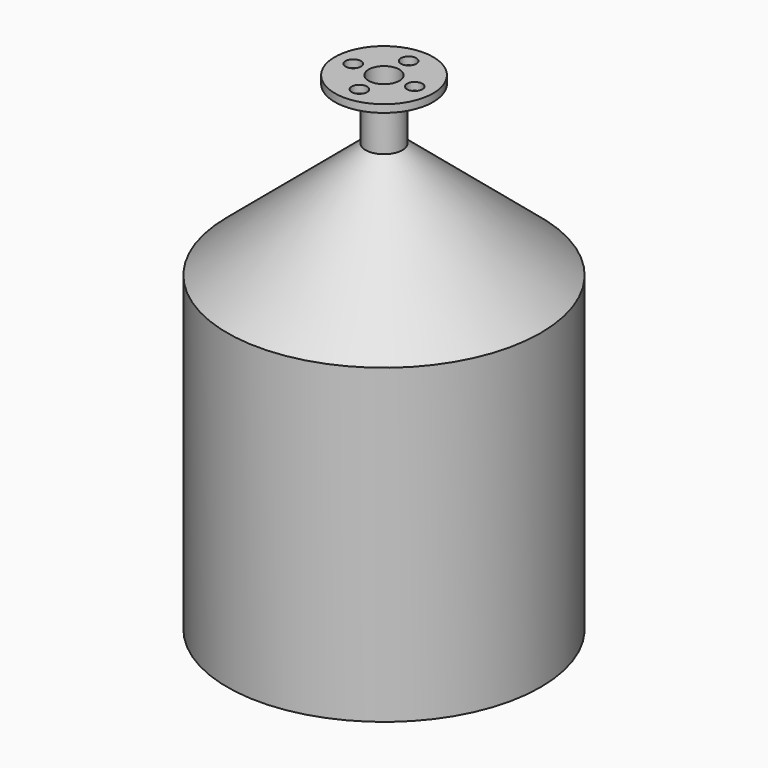
from build123d import *

# Parameters (mm, degrees)
F2_R     = 32
F2_R_2   = 12
F3_DEPTH = 5
F4_R     = 5
F5_DEPTH = 5


with BuildPart() as f1:
    # F0 (on Front) → F1 (revolve)
    with BuildSketch(Plane.XZ):
        Polygon((-100, 0), (-100, 200), (-10, 275.518966806), (-10, 315.518966806), (-12, 315.518966806), (-12, 276.4515821223), (-102, 200.9326153163), (-102, -2), (0, -2), (0, 0), align=None)
    revolve(axis=Axis((0, 0, 120), (0, 0, 1)))

    # F2 (on face) → F3 (join)
    with BuildSketch(Plane.XY.offset(315.518966806)):
        Circle(F2_R)
        Circle(F2_R_2, mode=Mode.SUBTRACT)
    extrude(amount=-F3_DEPTH)

    # F4 (on face) → F5 (cut, through all)
    with BuildSketch(Plane.XY.offset(315.518966806)):
        with Locations((0, 20)):
            Circle(F4_R)
        with Locations((-20, 0)):
            Circle(F4_R)
        with Locations((0, -20)):
            Circle(F4_R)
        with Locations((20, 0)):
            Circle(F4_R)
    extrude(amount=-F5_DEPTH, mode=Mode.SUBTRACT)


solid = f1.part
